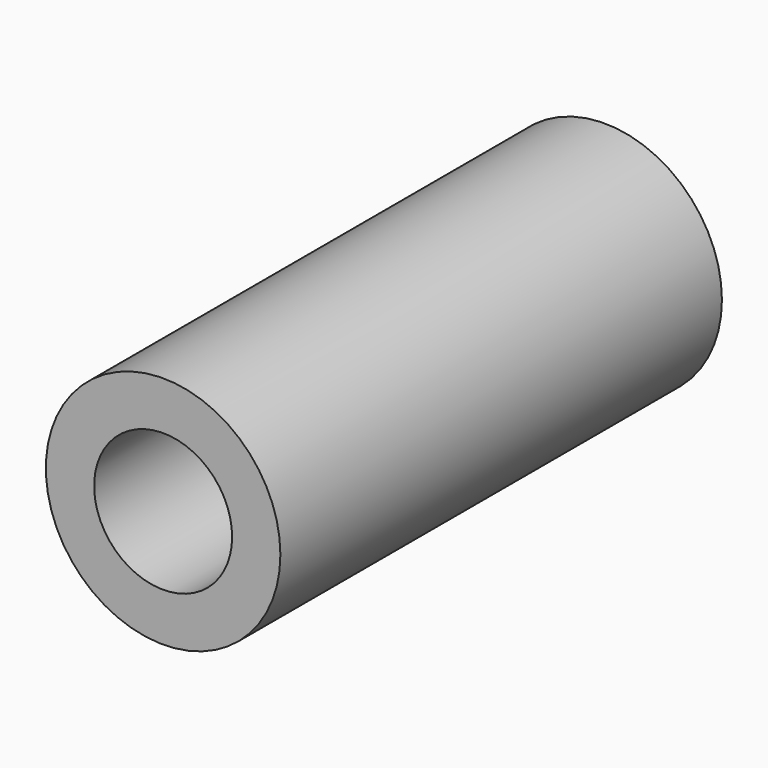
from build123d import *

# Parameters (mm, degrees)
F0_R     = 21.5867472132
F0_R_2   = 12.7
F1_DEPTH = 101.6


# Not quite as in the source:
# - the program builds the solid bodies; features that only make, move or delete a surface that nothing else refers to are left out


with BuildPart() as f1:
    # F0 (on Front) → F1 (new body)
    with BuildSketch(Plane.XZ):
        Circle(F0_R)
        Circle(F0_R_2, mode=Mode.SUBTRACT)
    extrude(amount=F1_DEPTH)


solid = f1.part
